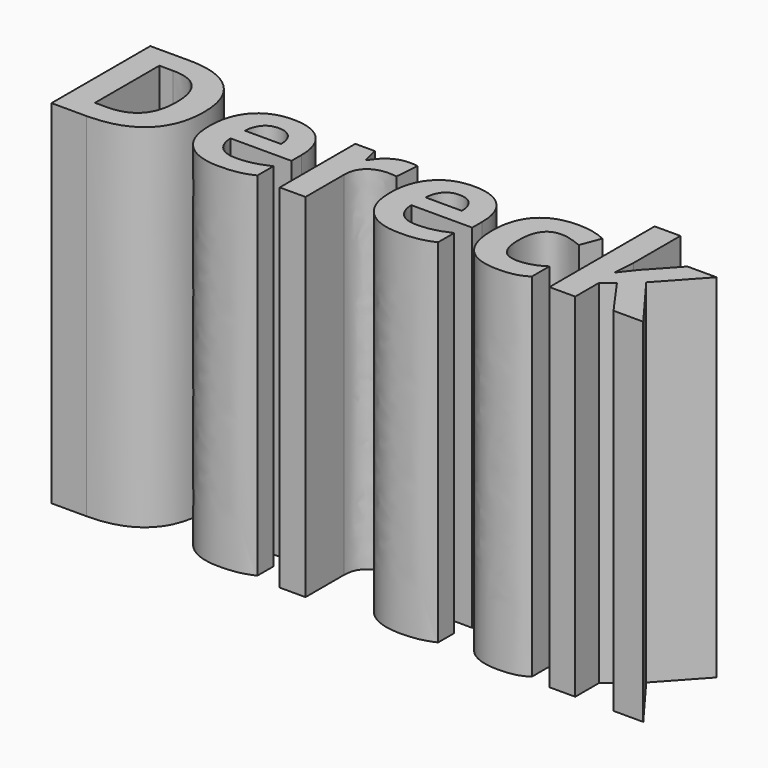
from build123d import *

# Parameters (mm, degrees)
F1_TEXT_SIZE = 54.0760863158
F0_DEPTH     = 110.1278904825


# Not quite as in the source:
# - Text() gives the source's letters only with a copy of the font that has no kerning and outlines rounded to 1/6400 em; it was checked with that copy


with BuildPart() as f0:
    # F1 (on Top) → F0 (new body)
    with BuildSketch(Plane.XY):
        with Locations((0, 0)):
            Text('Dereck', F1_TEXT_SIZE, font='Open Sans', font_style=FontStyle.BOLD, text_align=(TextAlign.LEFT, TextAlign.BOTTOM))
    extrude(amount=F0_DEPTH)


solid = f0.part
